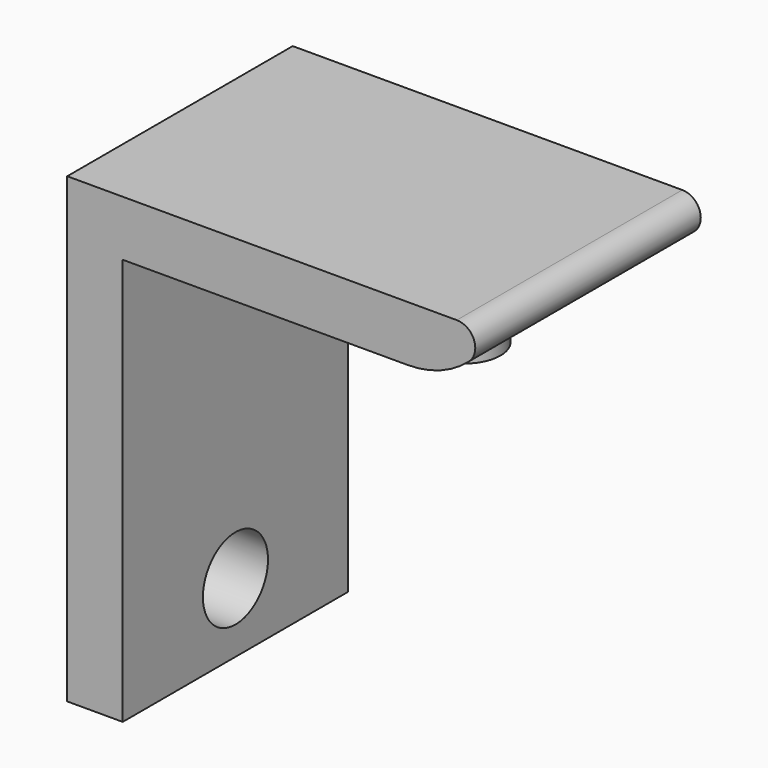
from build123d import *

# Parameters (mm, degrees)
F0_W        = 4.76
F0_H        = 15.24
F0_W_2      = 15.24
F0_R        = 1.95
F1_DEPTH    = 3
F2_DEPTH    = 3
F3_W        = 15.24
F3_H        = 22
F3_R        = 2.2
F3_H_2      = 3
F4_DEPTH    = 3
F5_T1_DEPTH = 38.1528784748
F6_R        = 1


# Not quite as in the source:
# - a fillet or chamfer that OpenCascade refuses, or shapes differently, is made with other operations: its cross-section is extruded or revolved along the edge and cut away or added
# - a feature names something its author has since deleted; it is built from what else it names


with BuildPart() as f1:
    # F0 (on Top) → F1 (new body)
    with BuildSketch(Plane.XY):
        with Locations((-7.62, 0)):
            Rectangle(F0_W, F0_H)
        with Locations((2.38, 0)):
            Rectangle(F0_W_2, F0_H)
        with Locations((2.38, 0)):
            Circle(F0_R, mode=Mode.SUBTRACT)
        with Locations((2.38, 0)):
            Circle(F0_R)
    extrude(amount=F1_DEPTH)

    # F0 (on Top) → F2 (join)
    with BuildSketch(Plane.XY):
        with Locations((2.38, 0)):
            Circle(F0_R)
    extrude(amount=-F2_DEPTH)

    # F3 (on face) → F4 (join)
    with BuildSketch(Plane(origin=(-10, 0, 0), x_dir=(0, -1, 0), z_dir=(-1, 0, 0))):
        with Locations((0, -11)):
            Rectangle(F3_W, F3_H)
        with Locations((0, -18.2633977383)):
            Circle(F3_R, mode=Mode.SUBTRACT)
        with Locations((0, 1.5)):
            Rectangle(F3_W, F3_H_2)
    extrude(amount=F4_DEPTH)

    # F5: fillet of radius 5 on 1 edges, made by hand

    # F5_s2 → F5_t1 (cut)
    with BuildSketch(Plane.XZ.offset(-19.0764392374)):
        with BuildLine():
            ThreePointArc((5.417424305, 0), (8.1560370926, 0.8166998673), (10, 3))
            Line((10, 3), (10, 0))
            Line((10, 0), (5.417424305, 0))
        make_face()
    extrude(amount=F5_T1_DEPTH, mode=Mode.SUBTRACT)

    # F6
    f6_edges = [f1.edges().sort_by_distance(p)[0] for p in [
        (10, 0, 3),
    ]]
    fillet(f6_edges, radius=F6_R)


solid = f1.part
